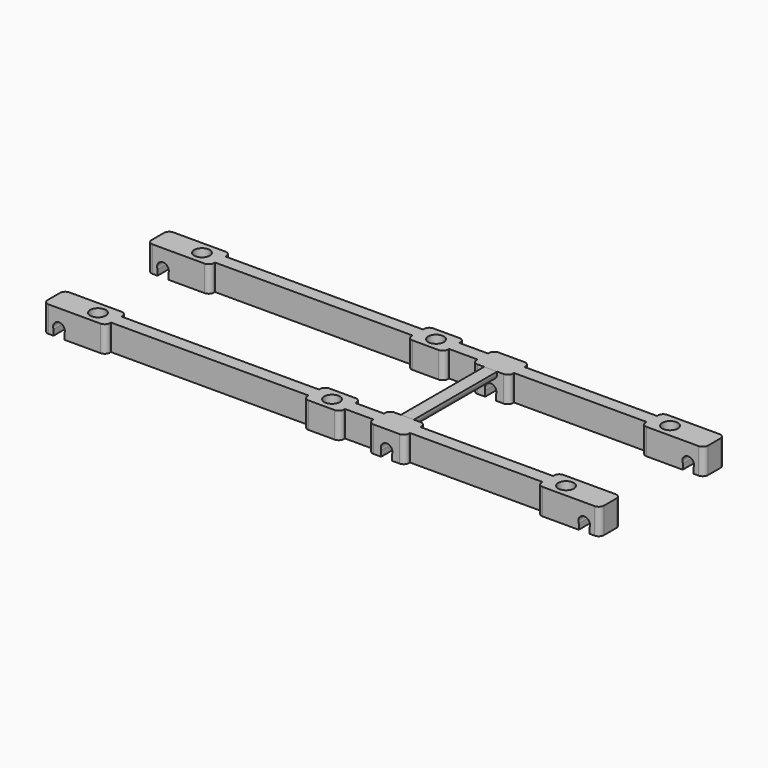
from build123d import *

# Parameters (mm, degrees)
F0_R     = 3
F1_DEPTH = 10
F3_DEPTH = 70
F4_R     = 2
F4_2_R   = 2
F5_W     = 5
F5_H     = 40
F6_DEPTH = 3
F7_R     = 2


with BuildPart() as f1:
    # F0 (on Top) → F1 (new body)
    with BuildSketch(Plane.XY):
        Polygon((83, 20), (107, 20), (107, 30), (83, 30), (83, 27.5), (32, 27.5), (32, 30), (18, 30), (18, 27.5), (7, 27.5), (7, 30), (-7, 30), (-7, 27.5), (-83, 27.5), (-83, 30), (-107, 30), (-107, 20), (-83, 20), (-83, 22.5), (-7, 22.5), (-7, 20), (7, 20), (7, 22.5), (18, 22.5), (18, 20), (32, 20), (32, 22.5), (83, 22.5), align=None)
        with Locations((-90, 25)):
            Circle(F0_R, mode=Mode.SUBTRACT)
        with Locations((0, 25)):
            Circle(F0_R, mode=Mode.SUBTRACT)
        with Locations((90, 25)):
            Circle(F0_R, mode=Mode.SUBTRACT)
    extrude(amount=F1_DEPTH)


with BuildPart() as f1b:
    # F0 (on Top) → F1, piece 2 (new body)
    with BuildSketch(Plane.XY):
        Polygon((83, -30), (107, -30), (107, -20), (83, -20), (83, -22.5), (32, -22.5), (32, -20), (18, -20), (18, -22.5), (7, -22.5), (7, -20), (-7, -20), (-7, -22.5), (-83, -22.5), (-83, -20), (-107, -20), (-107, -30), (-83, -30), (-83, -27.5), (-7, -27.5), (-7, -30), (7, -30), (7, -27.5), (18, -27.5), (18, -30), (32, -30), (32, -27.5), (83, -27.5), align=None)
        with Locations((-90, -25)):
            Circle(F0_R, mode=Mode.SUBTRACT)
        with Locations((0, -25)):
            Circle(F0_R, mode=Mode.SUBTRACT)
        with Locations((90, -25)):
            Circle(F0_R, mode=Mode.SUBTRACT)
    extrude(amount=F1_DEPTH)


with BuildPart() as f3_tool:
    # F2 (on face) → F3 (new body)
    with BuildSketch(Plane.XZ.offset(30)):
        with BuildLine():
            ThreePointArc((103.1, 2.1922252789), (103.2121821806, 2.5892080819), (103.25, 3))
            ThreePointArc((103.25, 3), (103.2121821806, 3.4107919181), (103.1, 3.8077747211))
            ThreePointArc((103.1, 3.8077747211), (101, 5.25), (98.9, 3.8077747211))
            ThreePointArc((98.9, 3.8077747211), (98.75, 3), (98.9, 2.1922252789))
            ThreePointArc((98.9, 2.1922252789), (101, 0.75), (103.1, 2.1922252789))
        make_face()
        with BuildLine():
            Line((103.1, -1.3476219028), (103.1, 2.1922252789))
            ThreePointArc((103.1, 2.1922252789), (101, 0.75), (98.9, 2.1922252789))
            Line((98.9, 2.1922252789), (98.9, -1.3476219028))
            Line((98.9, -1.3476219028), (103.1, -1.3476219028))
        make_face()
        with BuildLine():
            Line((-103.1, 2.1922252789), (-103.1, 0.0061060628))
            Line((-103.1, 0.0061060628), (-103.1, -2.6691132225))
            Line((-103.1, -2.6691132225), (-98.9, -2.6691132225))
            Line((-98.9, -2.6691132225), (-98.9, -0.0081721373))
            Line((-98.9, -0.0081721373), (-98.9, 2.1922252789))
            ThreePointArc((-98.9, 2.1922252789), (-101, 0.75), (-103.1, 2.1922252789))
        make_face()
        with BuildLine():
            ThreePointArc((-103.1, 3.8077747211), (-103.25, 3), (-103.1, 2.1922252789))
            ThreePointArc((-103.1, 2.1922252789), (-101, 0.75), (-98.9, 2.1922252789))
            ThreePointArc((-98.9, 2.1922252789), (-98.75, 3), (-98.9, 3.8077747211))
            ThreePointArc((-98.9, 3.8077747211), (-101, 5.25), (-103.1, 3.8077747211))
        make_face()
        with BuildLine():
            Line((22.9, 2.1922252789), (22.9, -4.3147648685))
            Line((22.9, -4.3147648685), (27.1, -4.3147648685))
            Line((27.1, -4.3147648685), (27.1, 2.1922252789))
            ThreePointArc((27.1, 2.1922252789), (25, 0.75), (22.9, 2.1922252789))
        make_face()
        with BuildLine():
            ThreePointArc((22.9, 3.8077747211), (22.75, 3), (22.9, 2.1922252789))
            ThreePointArc((22.9, 2.1922252789), (25, 0.75), (27.1, 2.1922252789))
            ThreePointArc((27.1, 2.1922252789), (27.25, 3), (27.1, 3.8077747211))
            ThreePointArc((27.1, 3.8077747211), (25, 5.25), (22.9, 3.8077747211))
        make_face()
    extrude(amount=-F3_DEPTH)


with BuildPart() as f1_1:
    add(f1.part)

    # F3: cut by f3_tool
    add(f3_tool.part, mode=Mode.SUBTRACT)

    # F4
    f4_edges = [f1_1.edges().sort_by_distance(p)[0] for p in [
        (-107, 20, 5),
        (-107, 30, 5),
        (-7, 20, 5),
        (-7, 30, 5),
        (18, 20, 5),
        (18, 30, 5),
        (83, 20, 5),
        (83, 30, 5),
        (-83, 20, 5),
        (-83, 30, 5),
        (7, 20, 5),
        (7, 30, 5),
        (32, 30, 5),
        (32, 20, 5),
        (107, 20, 5),
        (107, 30, 5),
    ]]
    fillet(f4_edges, radius=F4_R)


with BuildPart() as f1b_1:
    add(f1b.part)

    # F3: cut by f3_tool
    add(f3_tool.part, mode=Mode.SUBTRACT)

    # F4#2
    f4_2_edges = [f1b_1.edges().sort_by_distance(p)[0] for p in [
        (-83, -30, 5),
        (-83, -20, 5),
        (-107, -30, 5),
        (-107, -20, 5),
        (-7, -20, 5),
        (18, -20, 5),
        (-7, -30, 5),
        (18, -30, 5),
        (83, -20, 5),
        (83, -30, 5),
        (107, -30, 5),
        (107, -20, 5),
        (32, -20, 5),
        (32, -30, 5),
        (7, -30, 5),
        (7, -20, 5),
    ]]
    fillet(f4_2_edges, radius=F4_2_R)


with BuildPart() as f6:
    # F5 (on face) → F6 (new body)
    with BuildSketch(Plane.XY.offset(10)):
        with Locations((25, 0)):
            Rectangle(F5_W, F5_H)
    extrude(amount=-F6_DEPTH)

    # F7
    f7_edges = [f6.edges().sort_by_distance(p)[0] for p in [
        (27.5, 0, 7),
        (22.5, 0, 7),
    ]]
    fillet(f7_edges, radius=F7_R)


solid = Compound([f1_1.part, f1b_1.part, f6.part])
